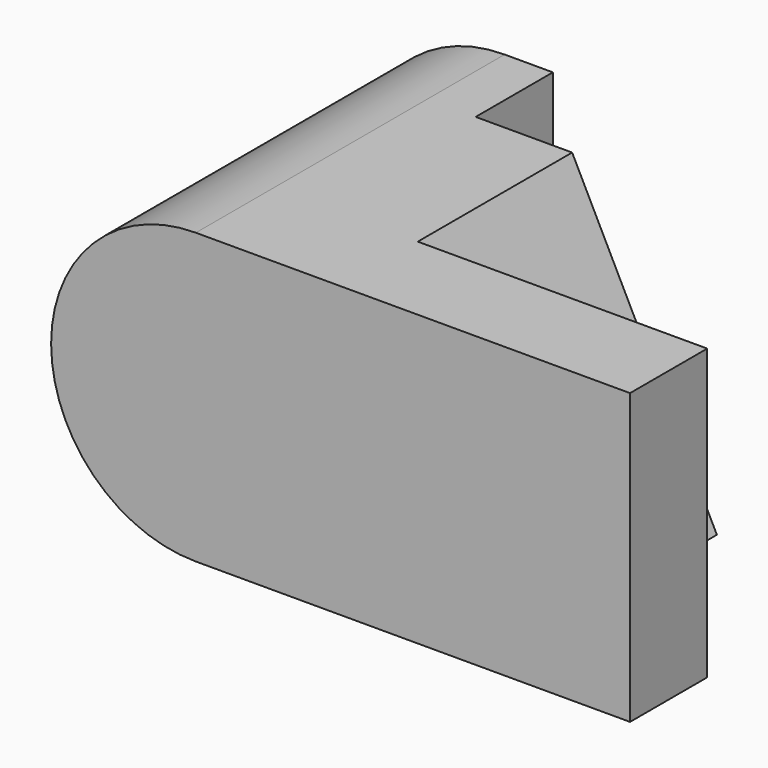
from build123d import *

# Parameters (mm, degrees)
F1_DEPTH = 30
F2_R     = 14.99999
F4_DEPTH = 20


# Not quite as in the source:
# - a fillet or chamfer is up to 0.001 mm smaller than in the source, because OpenCascade refuses the exact size


with BuildPart() as f1:
    # F0 (on Top) → F1 (new body)
    with BuildSketch(Plane.XY):
        Polygon((0, 40), (0, 0), (60, 0), (60, 10), (30, 10), (30, 30), (20, 30), (20, 40), align=None)
    extrude(amount=F1_DEPTH)

    # F2 (radius 15 in the source; OpenCascade refuses exactly that, so slightly less here)
    f2_edges = [f1.edges().sort_by_distance(p)[0] for p in [
        (0, 20, 30),
        (0, 20, 0),
    ]]
    fillet(f2_edges, radius=F2_R)

    # F3 (on face) → F4 (join)
    with BuildSketch(Plane(origin=(0, 10, 0), x_dir=(-1, 0, 0), z_dir=(0, 1, 0))):
        Polygon((-30, 0), (-30, 30), (-45, 0), align=None)
    extrude(amount=F4_DEPTH)


solid = f1.part
